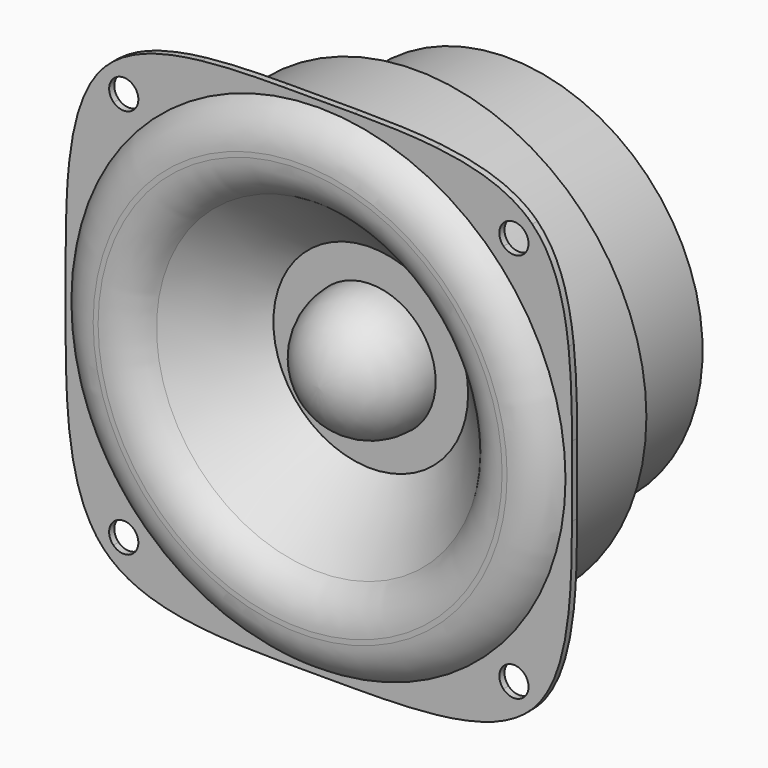
from build123d import *

# Parameters (mm, degrees)
F1_DEPTH  = 1
F2_R      = 35.5
F3_DEPTH  = 17.7
F4_R      = 30
F5_DEPTH  = 17.7
F6_R      = 25
F7_DEPTH  = 10
F8_R      = 10
F9_DEPTH  = 10
F10_R     = 9.99999
F11_R     = 38
F11_R_2   = 25
F12_DEPTH = 3.6
F13_SIZE  = 9.99999


# Not quite as in the source:
# - a fillet or chamfer that OpenCascade refuses, or shapes differently, is made with other operations: its cross-section is extruded or revolved along the edge and cut away or added
# - a fillet or chamfer is up to 0.001 mm smaller than in the source, because OpenCascade refuses the exact size
# - ends of sketch curves that miss each other by under 0.0002 mm in the source are joined


with BuildPart() as f1:
    # F0 (on Front) → F1 (new body)
    with BuildSketch(Plane.XZ):
        with BuildLine():
            Line((-31.6430284581, 31.6430284581), (-32.8804653252, 32.8804653252))
            add(Edge.make_bspline(
                [(-38.4634802867, 18.0779059693), (-37.7870588122, 24.2282956212), (-36.2701561309, 29.4907744999), (-32.8804653607, 32.8804652897)],
                knots=[0.809263962, 0.809263962, 0.809263962, 0.809263962, 0.875, 0.875, 0.875, 0.875], degree=3))
            ThreePointArc((-38.4634802867, 18.0779059693), (-35.411472746, 23.5005871833), (-31.6003565153, 28.4194909895))
            ThreePointArc((-31.6003565153, 28.4194909895), (-32.3018410876, 30.0222561796), (-31.6430284581, 31.6430284581))
        make_face()
        with BuildLine():
            add(Edge.make_bspline(
                [(-32.8804653607, 32.8804652897), (-29.4907745634, 36.2701561065), (-24.2282956474, 37.7870588046), (-18.077905986, 38.4634802832)],
                knots=[0.875, 0.875, 0.875, 0.875, 0.940736038, 0.940736038, 0.940736038, 0.940736038], degree=3))
            Line((-32.8804653252, 32.8804653252), (-31.6430284581, 31.6430284581))
            ThreePointArc((-31.6430284581, 31.6430284581), (-30.0222561796, 32.3018410876), (-28.4194909895, 31.6003565153))
            ThreePointArc((-28.4194909895, 31.6003565153), (-23.5005871834, 35.411472746), (-18.0779059693, 38.4634802867))
        make_face()
        with BuildLine():
            add(Edge.make_bspline(
                [(-38.4634802867, -18.0779059693), (-38.8960139665, -14.1450759683), (-38.9848843926, -9.8491893154), (-39, -5.4477534527)],
                knots=[0.690736038, 0.690736038, 0.690736038, 0.690736038, 0.7327705557, 0.7327705557, 0.7327705557, 0.7327705557], degree=3))
            ThreePointArc((-38.4634802867, -18.0779059693), (-35.411472746, -23.5005871834), (-31.6003565153, -28.4194909895))
            ThreePointArc((-31.6003565153, -28.4194909895), (-30.0222561796, -27.8022353132), (-28.4610479428, -28.4610479428))
            Line((-28.4610479428, -28.4610479428), (0, 0))
            Line((0, 0), (-28.4610479428, 28.4610479428))
            ThreePointArc((-28.4610479428, 28.4610479428), (-30.0222561796, 27.8022353132), (-31.6003565153, 28.4194909895))
            ThreePointArc((-31.6003565153, 28.4194909895), (-35.411472746, 23.5005871833), (-38.4634802867, 18.0779059693))
            add(Edge.make_bspline(
                [(-39, 5.4477534527), (-38.9848843926, 9.8491893154), (-38.8960139665, 14.1450759683), (-38.4634802867, 18.0779059693)],
                knots=[0.7672294443, 0.7672294443, 0.7672294443, 0.7672294443, 0.809263962, 0.809263962, 0.809263962, 0.809263962], degree=3))
            Line((-39, 5.4477534527), (-39, -2.257e-07))
            Line((-39, -2.257e-07), (-39, -5.4477534527))
        make_face()
        with BuildLine():
            ThreePointArc((28.4194909895, 31.6003565153), (23.5005871834, 35.411472746), (18.0779059693, 38.4634802867))
            add(Edge.make_bspline(
                [(5.4477534527, 39), (9.8491893154, 38.9848843926), (14.1450759683, 38.8960139665), (18.0779059693, 38.4634802867)],
                knots=[0.0172294443, 0.0172294443, 0.0172294443, 0.0172294443, 0.059263962, 0.059263962, 0.059263962, 0.059263962], degree=3))
            Line((5.4477534527, 39), (0, 39))
            Line((0, 39), (-5.4477534527, 39))
            add(Edge.make_bspline(
                [(-18.0779059693, 38.4634802867), (-14.1450759684, 38.8960139665), (-9.8491893154, 38.9848843926), (-5.4477534527, 39)],
                knots=[0.940736038, 0.940736038, 0.940736038, 0.940736038, 0.9827705557, 0.9827705557, 0.9827705557, 0.9827705557], degree=3))
            ThreePointArc((-18.0779059693, 38.4634802867), (-23.5005871834, 35.411472746), (-28.4194909895, 31.6003565153))
            ThreePointArc((-28.4194909895, 31.6003565153), (-27.9620942748, 30.885485492), (-27.8020382004, 30.0520382004))
            ThreePointArc((-27.8020382004, 30.0520382004), (-27.9733092523, 29.1910004776), (-28.4610479428, 28.4610479428))
            Line((-28.4610479428, 28.4610479428), (0, 0))
            Line((0, 0), (28.4610479428, 28.4610479428))
            ThreePointArc((28.4610479428, 28.4610479428), (27.8022353132, 30.0222561796), (28.4194909895, 31.6003565153))
        make_face()
        with BuildLine():
            ThreePointArc((31.6003565153, -28.4194909895), (35.411472746, -23.5005871834), (38.4634802867, -18.0779059693))
            add(Edge.make_bspline(
                [(39, -5.4477534527), (38.9848843926, -9.8491893154), (38.8960139665, -14.1450759683), (38.4634802867, -18.0779059693)],
                knots=[0.2672294443, 0.2672294443, 0.2672294443, 0.2672294443, 0.309263962, 0.309263962, 0.309263962, 0.309263962], degree=3))
            Line((39, -5.4477534527), (39, 6.014e-07))
            Line((39, 6.014e-07), (39, 5.4477534527))
            add(Edge.make_bspline(
                [(38.4634802867, 18.0779059693), (38.8960139665, 14.1450759683), (38.9848843926, 9.8491893154), (39, 5.4477534527)],
                knots=[0.190736038, 0.190736038, 0.190736038, 0.190736038, 0.2327705557, 0.2327705557, 0.2327705557, 0.2327705557], degree=3))
            ThreePointArc((38.4634802867, 18.0779059693), (35.411472746, 23.5005871834), (31.6003565153, 28.4194909895))
            ThreePointArc((31.6003565153, 28.4194909895), (30.0222561796, 27.8022353132), (28.4610479428, 28.4610479428))
            Line((28.4610479428, 28.4610479428), (0, 0))
            Line((0, 0), (28.4610479428, -28.4610479428))
            ThreePointArc((28.4610479428, -28.4610479428), (30.0222561796, -27.8022353132), (31.6003565153, -28.4194909895))
        make_face()
        with BuildLine():
            add(Edge.make_bspline(
                [(18.0779059693, -38.4634802867), (14.1450759683, -38.8960139665), (9.8491893154, -38.9848843926), (5.4477534527, -39)],
                knots=[0.440736038, 0.440736038, 0.440736038, 0.440736038, 0.4827705557, 0.4827705557, 0.4827705557, 0.4827705557], degree=3))
            ThreePointArc((18.0779059693, -38.4634802867), (23.5005871834, -35.411472746), (28.4194909895, -31.6003565153))
            ThreePointArc((28.4194909895, -31.6003565153), (27.8022353132, -30.0222561796), (28.4610479428, -28.4610479428))
            Line((28.4610479428, -28.4610479428), (0, 0))
            Line((0, 0), (-28.4610479428, -28.4610479428))
            ThreePointArc((-28.4610479428, -28.4610479428), (-27.9733092523, -29.1910004776), (-27.8020382004, -30.0520382004))
            ThreePointArc((-27.8020382004, -30.0520382004), (-27.9620942748, -30.885485492), (-28.4194909895, -31.6003565153))
            ThreePointArc((-28.4194909895, -31.6003565153), (-23.5005871834, -35.411472746), (-18.0779059693, -38.4634802867))
            add(Edge.make_bspline(
                [(-5.4477534527, -39), (-9.8491893154, -38.9848843926), (-14.1450759683, -38.8960139665), (-18.0779059693, -38.4634802867)],
                knots=[0.5172294443, 0.5172294443, 0.5172294443, 0.5172294443, 0.559263962, 0.559263962, 0.559263962, 0.559263962], degree=3))
            Line((-5.4477534527, -39), (-6.496e-07, -39))
            Line((-6.496e-07, -39), (5.4477534527, -39))
        make_face()
        with BuildLine():
            add(Edge.make_bspline(
                [(32.8804653252, -32.8804653252), (29.4907745274, -36.2701561229), (24.2282956212, -37.7870588122), (18.0779059693, -38.4634802867)],
                knots=[0.375, 0.375, 0.375, 0.375, 0.440736038, 0.440736038, 0.440736038, 0.440736038], degree=3))
            Line((32.8804653252, -32.8804653252), (31.6430284581, -31.6430284581))
            ThreePointArc((31.6430284581, -31.6430284581), (30.0222561796, -32.3018410876), (28.4194909895, -31.6003565153))
            ThreePointArc((28.4194909895, -31.6003565153), (23.5005871834, -35.411472746), (18.0779059693, -38.4634802867))
        make_face()
        with BuildLine():
            Line((31.6430284581, -31.6430284581), (32.8804653252, -32.8804653252))
            add(Edge.make_bspline(
                [(38.4634802867, -18.0779059693), (37.7870588122, -24.2282956212), (36.2701561229, -29.4907745274), (32.8804653252, -32.8804653252)],
                knots=[0.309263962, 0.309263962, 0.309263962, 0.309263962, 0.375, 0.375, 0.375, 0.375], degree=3))
            ThreePointArc((38.4634802867, -18.0779059693), (35.411472746, -23.5005871834), (31.6003565153, -28.4194909895))
            ThreePointArc((31.6003565153, -28.4194909895), (32.1191879541, -29.1635609099), (32.3020382004, -30.0520382004))
            ThreePointArc((32.3020382004, -30.0520382004), (32.1307671486, -30.9130759232), (31.6430284581, -31.6430284581))
        make_face()
        with BuildLine():
            Line((-31.6430284581, -31.6430284581), (-32.8804653252, -32.8804653252))
            add(Edge.make_bspline(
                [(-18.0779059693, -38.4634802867), (-24.2282956212, -37.7870588122), (-29.4907744533, -36.2701561443), (-32.8804653252, -32.8804653252)],
                knots=[0.559263962, 0.559263962, 0.559263962, 0.559263962, 0.625, 0.625, 0.625, 0.625], degree=3))
            ThreePointArc((-18.0779059693, -38.4634802867), (-23.5005871834, -35.411472746), (-28.4194909895, -31.6003565153))
            ThreePointArc((-28.4194909895, -31.6003565153), (-30.0222561796, -32.3018410876), (-31.6430284581, -31.6430284581))
        make_face()
        with BuildLine():
            add(Edge.make_bspline(
                [(-32.8804652296, -32.8804654207), (-36.2701560789, -29.4907746242), (-37.7870587922, -24.2282957051), (-38.4634802779, -18.0779060371)],
                knots=[0.625, 0.625, 0.625, 0.625, 0.690736038, 0.690736038, 0.690736038, 0.690736038], degree=3))
            Line((-32.8804652296, -32.8804654207), (-31.6430284581, -31.6430284581))
            ThreePointArc((-31.6430284581, -31.6430284581), (-32.3018410876, -30.0222561796), (-31.6003565153, -28.4194909895))
            ThreePointArc((-31.6003565153, -28.4194909895), (-35.411472746, -23.5005871834), (-38.4634802779, -18.0779060371))
        make_face()
        with BuildLine():
            Line((31.6430284581, 31.6430284581), (32.8804653252, 32.8804653252))
            add(Edge.make_bspline(
                [(18.0779059693, 38.4634802867), (24.2282956212, 37.7870588122), (29.4907744654, 36.2701561408), (32.8804653252, 32.8804653252)],
                knots=[0.059263962, 0.059263962, 0.059263962, 0.059263962, 0.125, 0.125, 0.125, 0.125], degree=3))
            ThreePointArc((18.0779059693, 38.4634802867), (23.5005871834, 35.411472746), (28.4194909895, 31.6003565153))
            ThreePointArc((28.4194909895, 31.6003565153), (30.0222561796, 32.3018410876), (31.6430284581, 31.6430284581))
        make_face()
        with BuildLine():
            add(Edge.make_bspline(
                [(32.8804652452, 32.8804654051), (36.2701560861, 29.4907746085), (37.7870587955, 24.2282956914), (38.4634802794, 18.077906026)],
                knots=[0.125, 0.125, 0.125, 0.125, 0.190736038, 0.190736038, 0.190736038, 0.190736038], degree=3))
            Line((32.8804652452, 32.8804654051), (31.6430284581, 31.6430284581))
            ThreePointArc((31.6430284581, 31.6430284581), (32.1307671486, 30.9130759232), (32.3020382004, 30.0520382004))
            ThreePointArc((32.3020382004, 30.0520382004), (32.1191879541, 29.1635609099), (31.6003565153, 28.4194909895))
            ThreePointArc((31.6003565153, 28.4194909895), (35.411472746, 23.5005871834), (38.4634802794, 18.077906026))
        make_face()
    extrude(amount=-F1_DEPTH)

    # F2 (on face) → F3 (join)
    with BuildSketch(Plane(origin=(0, 1, 0), x_dir=(-1, 0, 0), z_dir=(0, 1, 0))):
        Circle(F2_R)
    extrude(amount=F3_DEPTH)

    # F4 (on face) → F5 (join)
    with BuildSketch(Plane(origin=(0, 18.7, 0), x_dir=(-1, 0, 0), z_dir=(0, 1, 0))):
        Circle(F4_R)
    extrude(amount=F5_DEPTH)

    # F6 (on face) → F7 (cut)
    with BuildSketch(Plane.XZ):
        Circle(F6_R)
    extrude(amount=-F7_DEPTH, mode=Mode.SUBTRACT)

    # F8 (on face) → F9 (join)
    with BuildSketch(Plane.XZ.offset(-10)):
        Circle(F8_R)
    extrude(amount=F9_DEPTH)

    # F10 (radius 10 in the source; OpenCascade refuses exactly that, so slightly less here)
    f10_edges = [f1.edges().sort_by_distance(p)[0] for p in [
        (-10, 0, 0),
    ]]
    fillet(f10_edges, radius=F10_R)

    # F11 (on face) → F12 (join)
    with BuildSketch(Plane.XZ):
        Circle(F11_R)
        Circle(F11_R_2, mode=Mode.SUBTRACT)
    extrude(amount=F12_DEPTH)

    # F13 (size 10 in the source; OpenCascade refuses exactly that, so slightly less here)
    f13_edges = [f1.edges().sort_by_distance(p)[0] for p in [
        (-25, 10, 0),
    ]]
    chamfer(f13_edges, length=F13_SIZE)

    # F14: fillet of radius 7 on 2 edges, made by hand

    # F14_s1 → F14_t2 (revolve, cut)
    with BuildSketch(Plane.XY):
        with BuildLine():
            ThreePointArc((31.8811765837, -3.6), (35.4308244535, -2.6332412516), (38, 0))
            Line((38, 0), (38.1223764683, -0.068))
            ThreePointArc((38.1223764683, -0.068), (38.14, -1.8), (38.14, -3.6))
            Line((38.14, -3.6), (38, -3.74))
            Line((38, -3.74), (31.8811765837, -3.74))
            Line((31.8811765837, -3.74), (31.8811765837, -3.6))
        make_face()
    revolve(axis=Axis((0, -3.6, 0), (0, -1, 0)), mode=Mode.SUBTRACT)

    # F14_s3 → F14_t4 (revolve, cut)
    with BuildSketch(Plane.XY):
        with BuildLine():
            ThreePointArc((25, 1e-05), (27.569176173, -2.633238351), (31.1188289729, -3.6))
            Line((31.1188289729, -3.6), (31.1188289729, -3.74))
            Line((31.1188289729, -3.74), (25, -3.74))
            Line((25, -3.74), (24.86, -3.6))
            ThreePointArc((24.86, -3.6), (24.86, -1.799995), (24.8776234205, -0.0679898))
            Line((24.8776234205, -0.0679898), (25, 1e-05))
        make_face()
    revolve(axis=Axis((0, -3.6, 0), (0, -1, 0)), mode=Mode.SUBTRACT)


solid = f1.part
